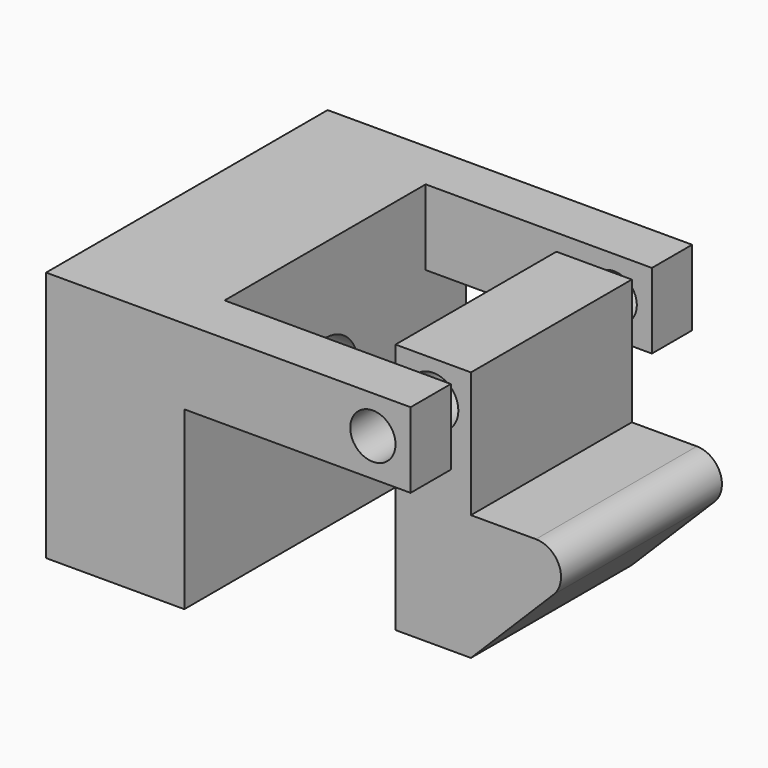
from build123d import *

# Parameters (mm, degrees)
F1_DEPTH       = 8
F2_R           = 1
F3_DEPTH       = 8.001
F4_R           = 1.65
F5_DEPTH       = 2
F6_R           = 1.25
F7_DEPTH       = 8
F8_R           = 0.9
F9_DEPTH       = 1
F9_DEPTH_BACK  = 9
F11_DEPTH      = 2
F12_W          = 13.5
F12_H          = 3
F13_DEPTH      = 2
F14_W          = 14
F14_H          = 10
F15_DEPTH      = 1
F15_DEPTH_BACK = 4.5
F17_R          = 1.65
F18_DEPTH      = 3
F20_DEPTH      = 3
F21_R          = 0.9
F22_DEPTH      = 14.001


with BuildPart() as f1:
    # F0 (on Front) → F1 (new body)
    with BuildSketch(Plane.XZ):
        with BuildLine():
            Line((0, 10), (0, 0))
            Line((0, 0), (3, 0))
            Line((3, 0), (6.2928932188, 3.2928932188))
            ThreePointArc((6.2928932188, 3.2928932188), (6.5096659701, 4.3826834324), (5.5857864376, 5))
            Line((5.5857864376, 5), (3, 5))
            Line((3, 5), (3, 10))
            Line((3, 10), (0, 10))
        make_face()
    extrude(amount=F1_DEPTH)

    # F2 (on face) → F3 (cut, through all)
    with BuildSketch(Plane.XZ.offset(8)):
        with Locations((1.5, 8.5)):
            Circle(F2_R)
    extrude(amount=-F3_DEPTH, mode=Mode.SUBTRACT)

    # F4 (on face) → F5 (cut)
    with BuildSketch(Plane(origin=(0, 0, 0), x_dir=(0, -1, 0), z_dir=(-1, 0, 0))):
        with Locations((4, 5)):
            Circle(F4_R)
    extrude(amount=-F5_DEPTH, mode=Mode.SUBTRACT)


with BuildPart() as f7:
    # F6 (on face) → F7 (new body)
    with BuildSketch(Plane(origin=(2, 0, 0), x_dir=(0, -1, 0), z_dir=(-1, 0, 0))):
        with Locations((4, 5)):
            Circle(F6_R)
    extrude(amount=F7_DEPTH)

    # F20 (add): a face of the model
    f20_faces = [f7.faces().sort_by_distance(p)[0] for p in [
        (-6, -4, 5),
    ]]
    extrude(f20_faces, amount=F20_DEPTH)


with BuildPart() as f9:
    # F8 (on face) → F9 (new body, two sides)
    with BuildSketch(Plane(origin=(0, 0, 0), x_dir=(-1, 0, 0), z_dir=(0, 1, 0))) as f9_sk:
        with Locations((-1.5, 8.5)):
            Circle(F8_R)
    extrude(amount=F9_DEPTH)
    extrude(f9_sk.sketch, amount=-F9_DEPTH_BACK)

    # F10 (on face) → F11 (join)
    with BuildSketch(Plane.XZ.offset(9)):
        Polygon((3, 10), (1.5, 10), (-10.5, 10), (-10.5, 7), (3, 7), align=None)
    extrude(amount=F11_DEPTH)

    # F12 (on face) → F13 (join)
    with BuildSketch(Plane(origin=(0, 1, 0), x_dir=(-1, 0, 0), z_dir=(0, 1, 0))):
        with Locations((3.75, 8.5)):
            Rectangle(F12_W, F12_H)
    extrude(amount=F13_DEPTH)

    # F14 (on face) → F15 (join, two sides)
    with BuildSketch(Plane(origin=(-10.5, 0, 0), x_dir=(0, -1, 0), z_dir=(-1, 0, 0))) as f15_sk:
        with Locations((4, 5)):
            Rectangle(F14_W, F14_H)
    extrude(amount=F15_DEPTH)
    extrude(f15_sk.sketch, amount=-F15_DEPTH_BACK)

    # F16: union 


with BuildPart() as f18:
    # F17 (on face) → F18 (new body)
    with BuildSketch(Plane(origin=(-6, 0, 0), x_dir=(0, -1, 0), z_dir=(-1, 0, 0))):
        with Locations((4, 5)):
            Circle(F17_R)
    extrude(amount=F18_DEPTH)


with BuildPart() as f9_1:
    add(f9.part)

    # F19: cut F18
    add(f18.part, mode=Mode.SUBTRACT)

    # F21 (on face) → F22 (cut, through all)
    with BuildSketch(Plane.XZ.offset(11)):
        with Locations((1.5, 8.5)):
            Circle(F21_R)
    extrude(amount=-F22_DEPTH, mode=Mode.SUBTRACT)


solid = Compound([f1.part, f7.part, f9_1.part])
